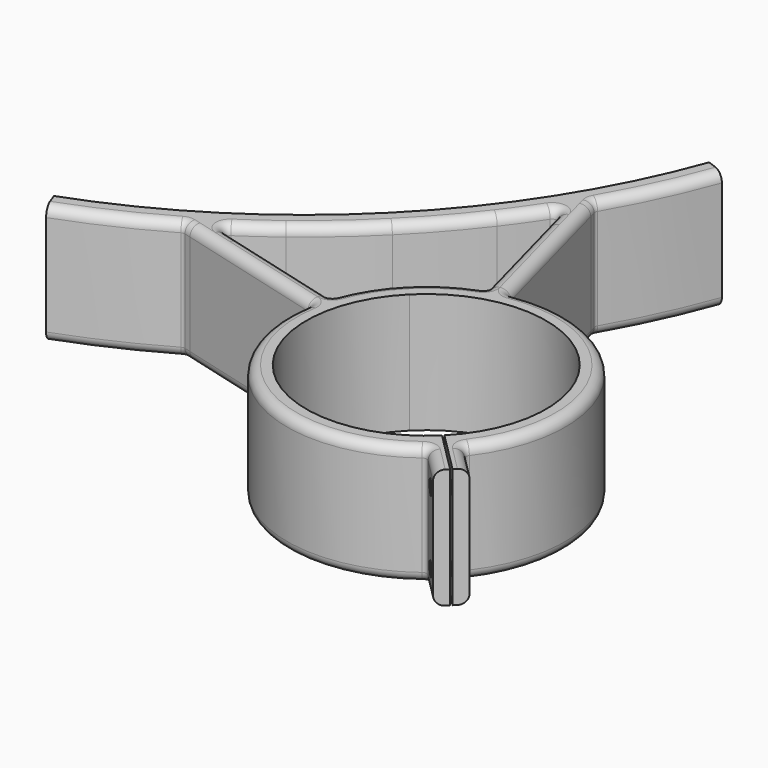
from build123d import *

# Parameters (mm, degrees)
F1_DEPTH = 31.75
F3_D     = 3.7973
F4_R     = 2.54
F5_R     = 2.53999


# Not quite as in the source:
# - a fillet or chamfer is up to 0.001 mm smaller than in the source, because OpenCascade refuses the exact size


with BuildPart() as f1:
    # F0 (on Top) → F1 (new body)
    with BuildSketch(Plane.XY):
        with BuildLine():
            ThreePointArc((114.0492527376, -114.0492527376), (86.6610538303, -136.0306062952), (55.164428917, -151.5630228066))
            Line((55.164428917, -151.5630228066), (56.9018912451, -156.3366613202))
            ThreePointArc((56.9018912451, -156.3366613202), (70.1800859457, -150.8434036896), (82.9347342482, -144.2248479118))
            ThreePointArc((82.9347342482, -144.2248479118), (83.4031486221, -144.0665225534), (83.8965240099, -144.0990751499))
            Line((83.8965240099, -144.0990751499), (85.582891778, -144.5509360315))
            Line((85.582891778, -144.5509360315), (95.6874921305, -147.2584555358))
            ThreePointArc((95.6874921305, -147.2584555358), (95.9820494866, -146.0228067737), (96.2994426244, -144.7928256782))
            ThreePointArc((96.2994426244, -144.7928256782), (96.6395626519, -143.5689342344), (97.0022928796, -142.3515523382))
            Line((97.0022928796, -142.3515523382), (92.1497093549, -141.0513065016))
            ThreePointArc((92.1497093549, -141.0513065016), (91.2248889076, -140.0285072053), (91.7778155305, -138.7653035757))
            ThreePointArc((91.7778155305, -138.7653035757), (96.4761342884, -135.5408883428), (101.0612739482, -132.1574659562))
            ThreePointArc((101.0612739482, -132.1574659562), (109.5919219903, -125.1742287153), (117.641355186, -117.641355186))
            Line((117.641355186, -117.641355186), (114.0492527376, -114.0492527376))
        make_face()
        with BuildLine():
            Line((140.0919954887, -140.0919954887), (136.4998930403, -136.4998930403))
            ThreePointArc((136.4998930403, -136.4998930403), (131.6088210682, -142.5539388185), (128.0991403187, -149.5006068225))
            ThreePointArc((128.0991403187, -149.5006068225), (127.4905756782, -150.1811446763), (126.582733391, -150.277607485))
            Line((126.582733391, -150.277607485), (97.0022928796, -142.3515523382))
            ThreePointArc((97.0022928796, -142.3515523382), (96.6395626519, -143.5689342344), (96.2994426244, -144.7928256782))
            ThreePointArc((96.2994426244, -144.7928256782), (95.9820494866, -146.0228067737), (95.6874921305, -147.2584555358))
            Line((95.6874921305, -147.2584555358), (125.2679326418, -155.1845106826))
            ThreePointArc((125.2679326418, -155.1845106826), (126.0059157209, -155.7219710691), (126.1926792325, -156.6156164589))
            ThreePointArc((126.1926792325, -156.6156164589), (143.5949774582, -194.1248324168), (184.8804836983, -191.8252150986))
            ThreePointArc((184.8804836983, -191.8252150986), (185.7356106095, -191.5677972619), (186.5487799279, -191.9369336005))
            Line((186.5487799279, -191.9369336005), (193.075506603, -198.4636602756))
            Line((193.075506603, -198.4636602756), (195.5899783169, -195.9491885617))
            Line((195.5899783169, -195.9491885617), (188.40577342, -188.7649836649))
            Line((188.40577342, -188.7649836649), (184.8129525396, -185.1721627845))
            ThreePointArc((184.8129525396, -185.1721627845), (140.0023718177, -184.9032932057), (140.0919954887, -140.0919954887))
        make_face()
        with BuildLine():
            Line((156.3366613202, -56.9018912451), (151.5630228066, -55.164428917))
            ThreePointArc((151.5630228066, -55.164428917), (136.0306062952, -86.6610538303), (114.0492527376, -114.0492527376))
            Line((114.0492527376, -114.0492527376), (117.641355186, -117.641355186))
            ThreePointArc((117.641355186, -117.641355186), (125.1742287153, -109.5919219903), (132.1574659562, -101.0612739482))
            ThreePointArc((132.1574659562, -101.0612739482), (135.5408883428, -96.4761342884), (138.7653035757, -91.7778155305))
            ThreePointArc((138.7653035757, -91.7778155305), (140.0285072053, -91.2248889076), (141.0513065016, -92.1497093549))
            Line((141.0513065016, -92.1497093549), (142.3515523382, -97.0022928796))
            Line((142.3515523382, -97.0022928796), (150.277607485, -126.582733391))
            ThreePointArc((150.277607485, -126.582733391), (150.1811446763, -127.4905756782), (149.5006068225, -128.0991403187))
            ThreePointArc((149.5006068225, -128.0991403187), (142.5539388185, -131.6088210682), (136.4998930403, -136.4998930403))
            Line((136.4998930403, -136.4998930403), (140.0919954887, -140.0919954887))
            ThreePointArc((140.0919954887, -140.0919954887), (184.9032932057, -140.0023718177), (185.1721627845, -184.8129525396))
            Line((185.1721627845, -184.8129525396), (188.7649836649, -188.40577342))
            Line((188.7649836649, -188.40577342), (195.9491885617, -195.5899783169))
            Line((195.9491885617, -195.5899783169), (198.4636602756, -193.075506603))
            Line((198.4636602756, -193.075506603), (191.9369336005, -186.5487799279))
            ThreePointArc((191.9369336005, -186.5487799279), (191.5677972619, -185.7356106095), (191.8252150986, -184.8804836983))
            ThreePointArc((191.8252150986, -184.8804836983), (194.1248324168, -143.5949774582), (156.6156164589, -126.1926792325))
            ThreePointArc((156.6156164589, -126.1926792325), (155.7219710691, -126.0059157209), (155.1845106826, -125.2679326418))
            Line((155.1845106826, -125.2679326418), (147.2584555358, -95.6874921305))
            Line((147.2584555358, -95.6874921305), (144.5509360315, -85.582891778))
            Line((144.5509360315, -85.582891778), (144.0990751499, -83.8965240099))
            ThreePointArc((144.0990751499, -83.8965240099), (144.0665225534, -83.4031486221), (144.2248479118, -82.9347342482))
            ThreePointArc((144.2248479118, -82.9347342482), (150.8434036896, -70.1800859457), (156.3366613202, -56.9018912451))
        make_face()
    extrude(amount=F1_DEPTH)

    # F3 (through all)
    with Locations(Plane(origin=(-2.6940768363, -2.6940768363, 0), x_dir=(0.7071067812, -0.7071067812, 0), z_dir=(-0.7071067812, -0.7071067812, 0))):
        with Locations((272.2449073091, 25.4), (272.2449073091, 6.35)):
            Hole(F3_D / 2)

    # F4
    f4_edges = [f1.edges().sort_by_distance(p)[0] for p in [
        (143.594977, -194.124832, 31.75),
        (194.124832, -143.594977, 31.75),
        (143.594977, -194.124832, 0),
        (194.124832, -143.594977, 0),
    ]]
    fillet(f4_edges, radius=F4_R)

    # F5 (radius 2.54 in the source; OpenCascade refuses exactly that, so slightly less here)
    f5_edges = [f1.edges().sort_by_distance(p)[0] for p in [
        (145.664457, -109.366221, 31.75),
        (109.366221, -145.664457, 0),
    ]]
    fillet(f5_edges, radius=F5_R)


solid = f1.part
